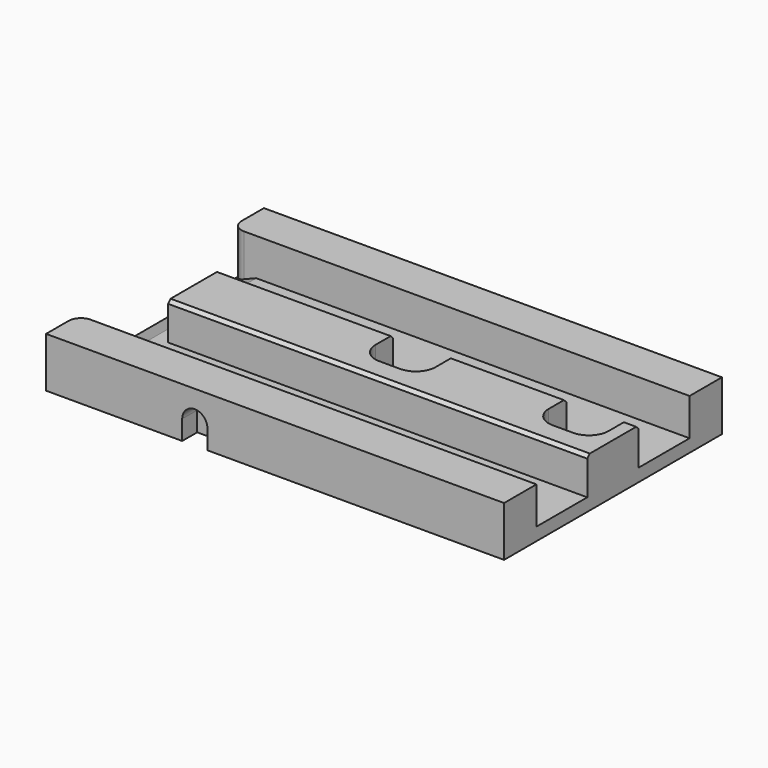
from build123d import *

# Parameters (mm, degrees)
F0_W      = 185.72
F0_H      = 110.42
F1_DEPTH  = 5.2
F3_DEPTH  = 110.42
F4_W      = 185.72
F4_H      = 16.4
F5_DEPTH  = 20.3
F6_W      = 24.4
F6_H      = 17
F6_W_2    = 24.3
F7_DEPTH  = 15.1
F8_R      = 8
F9_R      = 8
F10_R     = 5
F11_SIZE  = 1.3
F14_DEPTH = 7.6
F16_DEPTH = 7.6
F17_DEPTH = 20.301


with BuildPart() as f1:
    # F0 (on Top) → F1 (new body)
    with BuildSketch(Plane.XY):
        with Locations((-8.2149282098, -9.908063139)):
            Rectangle(F0_W, F0_H)
    extrude(amount=F1_DEPTH)

    # F2 (on face) → F3 (cut, through all)
    with BuildSketch(Plane.XZ.offset(65.118063139)):
        Polygon((-91.0749282098, 5.2), (-101.0749282098, 5.2), (-101.0749282098, 1.2), align=None)
    extrude(amount=-F3_DEPTH, mode=Mode.SUBTRACT)

    # F4 (on face) → F5 (join)
    with BuildSketch(Plane(origin=(0, 0, 0), x_dir=(1, 0, 0), z_dir=(0, 0, -1))):
        with Locations((-8.2149282098, 56.918063139)):
            Rectangle(F4_W, F4_H)
        with Locations((-8.2149282098, -37.101936861)):
            Rectangle(F4_W, F4_H)
        Polygon((84.6450717902, 9.908063139), (84.6450717902, 22.958063139), (-85.3549282098, 22.958063139), (-85.3549282098, 9.908063139), (-85.3549282098, -3.141936861), (84.6450717902, -3.141936861), align=None)
    extrude(amount=-F5_DEPTH)

    # F6 (on face) → F7 (cut)
    with BuildSketch(Plane.XY.offset(20.3)):
        with Locations((-2.7149282098, -5.358063139)):
            Rectangle(F6_W, F6_H)
        with Locations((67.4950717902, -5.358063139)):
            Rectangle(F6_W_2, F6_H)
    extrude(amount=-F7_DEPTH, mode=Mode.SUBTRACT)

    # F8
    f8_edges = [f1.edges().sort_by_distance(p)[0] for p in [
        (-14.914928, -13.858063, 12.75),
    ]]
    fillet(f8_edges, radius=F8_R)

    # F9
    f9_edges = [f1.edges().sort_by_distance(p)[0] for p in [
        (9.485072, -13.858063, 12.75),
        (79.645072, -13.858063, 12.75),
        (55.345072, -13.858063, 12.75),
    ]]
    fillet(f9_edges, radius=F9_R)

    # F10
    f10_edges = [f1.edges().sort_by_distance(p)[0] for p in [
        (-101.074928, 28.901937, 10.75),
        (-101.074928, -48.718063, 10.75),
    ]]
    fillet(f10_edges, radius=F10_R)

    # F11
    f11_edges = [f1.edges().sort_by_distance(p)[0] for p in [
        (-50.134928, 3.141937, 20.3),
        (32.415072, 3.141937, 20.3),
        (82.145072, 3.141937, 20.3),
        (-0.354928, -22.958063, 20.3),
    ]]
    chamfer(f11_edges, length=F11_SIZE)

    # F13 (on face) → F14 (cut)
    with BuildSketch(Plane.XZ.offset(65.118063139)):
        with BuildLine():
            Line((-45.8749282098, 7.9100113362), (-45.8749282098, 0))
            Line((-45.8749282098, 0), (-40.7749282098, 0))
            Line((-40.7749282098, 0), (-40.7749282098, 2.8100113362))
            ThreePointArc((-40.7749282098, 2.8100113362), (-44.3811727938, 4.3037667522), (-45.8749282098, 7.9100113362))
        make_face()
        with BuildLine():
            Line((-40.7749282098, 2.8100113362), (-40.7749282098, 0))
            Line((-40.7749282098, 0), (-35.6749282098, 0))
            Line((-35.6749282098, 0), (-35.6749282098, 7.9100113362))
            ThreePointArc((-35.6749282098, 7.9100113362), (-37.1686836257, 4.3037667522), (-40.7749282098, 2.8100113362))
        make_face()
        with BuildLine():
            Line((-40.7749282098, 7.9100113362), (-45.8749282098, 7.9100113362))
            ThreePointArc((-45.8749282098, 7.9100113362), (-44.3811727938, 4.3037667522), (-40.7749282098, 2.8100113362))
            Line((-40.7749282098, 2.8100113362), (-40.7749282098, 7.9100113362))
        make_face()
        with BuildLine():
            ThreePointArc((-35.6749282098, 7.9100113362), (-40.7749282098, 13.0100113362), (-45.8749282098, 7.9100113362))
            Line((-45.8749282098, 7.9100113362), (-40.7749282098, 7.9100113362))
            Line((-40.7749282098, 7.9100113362), (-35.6749282098, 7.9100113362))
        make_face()
        with BuildLine():
            Line((-40.7749282098, 7.9100113362), (-40.7749282098, 2.8100113362))
            ThreePointArc((-40.7749282098, 2.8100113362), (-37.1686836257, 4.3037667522), (-35.6749282098, 7.9100113362))
            Line((-35.6749282098, 7.9100113362), (-40.7749282098, 7.9100113362))
        make_face()
    extrude(amount=-F14_DEPTH, mode=Mode.SUBTRACT)

    # F15 (on face) → F16 (cut)
    with BuildSketch(Plane(origin=(0, 45.301936861, 0), x_dir=(-1, 0, 0), z_dir=(0, 1, 0))):
        with BuildLine():
            Line((40.7749282098, 0), (45.8749282098, 0))
            Line((45.8749282098, 0), (45.8749282098, 7.9))
            ThreePointArc((45.8749282098, 7.9), (44.3811727938, 4.2937554159), (40.7749282098, 2.8))
            Line((40.7749282098, 2.8), (40.7749282098, 0))
        make_face()
        with BuildLine():
            Line((35.6749282098, 0), (40.7749282098, 0))
            Line((40.7749282098, 0), (40.7749282098, 2.8))
            ThreePointArc((40.7749282098, 2.8), (37.1686836257, 4.2937554159), (35.6749282098, 7.9))
            Line((35.6749282098, 7.9), (35.6749282098, 0))
        make_face()
        with BuildLine():
            ThreePointArc((40.7749282098, 2.8), (44.3811727938, 4.2937554159), (45.8749282098, 7.9))
            Line((45.8749282098, 7.9), (40.7749282098, 7.9))
            Line((40.7749282098, 7.9), (40.7749282098, 2.8))
        make_face()
        with BuildLine():
            ThreePointArc((35.6749282098, 7.9), (37.1686836257, 4.2937554159), (40.7749282098, 2.8))
            Line((40.7749282098, 2.8), (40.7749282098, 7.9))
            Line((40.7749282098, 7.9), (35.6749282098, 7.9))
        make_face()
        with BuildLine():
            Line((40.7749282098, 7.9), (45.8749282098, 7.9))
            ThreePointArc((45.8749282098, 7.9), (40.7749282098, 13), (35.6749282098, 7.9))
            Line((35.6749282098, 7.9), (40.7749282098, 7.9))
        make_face()
    extrude(amount=-F16_DEPTH, mode=Mode.SUBTRACT)

    # F12 (on face) → F17 (cut, through all)
    with BuildSketch(Plane(origin=(0, 0, 0), x_dir=(1, 0, 0), z_dir=(0, 0, -1))):
        with BuildLine():
            ThreePointArc((-0.9549282098, -1.951936861), (1.9795649321, -0.7364300029), (3.1950717902, 2.198063139))
            Line((3.1950717902, 2.198063139), (-0.7049282098, 2.198063139))
            ThreePointArc((-0.7049282098, 2.198063139), (-1.2971901643, 0.0614770771), (-2.9049282098, -1.4652686778))
            ThreePointArc((-2.9049282098, -1.4652686778), (-1.9598344144, -1.8284320516), (-0.9549282098, -1.951936861))
        make_face()
        with BuildLine():
            Line((-0.7049282098, 2.198063139), (3.1950717902, 2.198063139))
            ThreePointArc((3.1950717902, 2.198063139), (1.9795649321, 5.132556281), (-0.9549282098, 6.348063139))
            ThreePointArc((-0.9549282098, 6.348063139), (-1.9598344144, 6.2245583296), (-2.9049282098, 5.8613949558))
            ThreePointArc((-2.9049282098, 5.8613949558), (-1.2971901643, 4.334649201), (-0.7049282098, 2.198063139))
        make_face()
        with BuildLine():
            ThreePointArc((69.0750717902, -1.951936861), (72.0095649321, -0.7364300029), (73.2250717902, 2.198063139))
            Line((73.2250717902, 2.198063139), (69.3250717902, 2.198063139))
            ThreePointArc((69.3250717902, 2.198063139), (68.7328098357, 0.0614770771), (67.1250717902, -1.4652686778))
            ThreePointArc((67.1250717902, -1.4652686778), (68.0701655856, -1.8284320516), (69.0750717902, -1.951936861))
        make_face()
        with BuildLine():
            Line((69.3250717902, 2.198063139), (73.2250717902, 2.198063139))
            ThreePointArc((73.2250717902, 2.198063139), (72.0095649321, 5.132556281), (69.0750717902, 6.348063139))
            ThreePointArc((69.0750717902, 6.348063139), (68.0701655856, 6.2245583296), (67.1250717902, 5.8613949558))
            ThreePointArc((67.1250717902, 5.8613949558), (68.7328098357, 4.334649201), (69.3250717902, 2.198063139))
        make_face()
        with BuildLine():
            ThreePointArc((67.1250717902, -1.4652686778), (68.7328098357, 0.0614770771), (69.3250717902, 2.198063139))
            Line((69.3250717902, 2.198063139), (69.0750717902, 2.198063139))
            Line((69.0750717902, 2.198063139), (65.1750717902, 2.198063139))
            Line((65.1750717902, 2.198063139), (64.9250717902, 2.198063139))
            ThreePointArc((64.9250717902, 2.198063139), (65.5173337448, 0.0614770771), (67.1250717902, -1.4652686778))
        make_face()
        with BuildLine():
            Line((69.0750717902, 2.198063139), (69.3250717902, 2.198063139))
            ThreePointArc((69.3250717902, 2.198063139), (68.7328098357, 4.334649201), (67.1250717902, 5.8613949558))
            ThreePointArc((67.1250717902, 5.8613949558), (65.5173337448, 4.334649201), (64.9250717902, 2.198063139))
            Line((64.9250717902, 2.198063139), (65.1750717902, 2.198063139))
            Line((65.1750717902, 2.198063139), (69.0750717902, 2.198063139))
        make_face()
        with BuildLine():
            ThreePointArc((67.1250717902, 5.8613949558), (68.0701655856, 6.2245583296), (69.0750717902, 6.348063139))
            Line((69.0750717902, 6.348063139), (65.1750717902, 6.348063139))
            ThreePointArc((65.1750717902, 6.348063139), (66.1799779949, 6.2245583296), (67.1250717902, 5.8613949558))
        make_face()
        with BuildLine():
            Line((65.1750717902, -1.951936861), (69.0750717902, -1.951936861))
            ThreePointArc((69.0750717902, -1.951936861), (68.0701655856, -1.8284320516), (67.1250717902, -1.4652686778))
            ThreePointArc((67.1250717902, -1.4652686778), (66.1799779949, -1.8284320516), (65.1750717902, -1.951936861))
        make_face()
        with BuildLine():
            ThreePointArc((64.9250717902, 2.198063139), (65.5173337448, 4.334649201), (67.1250717902, 5.8613949558))
            ThreePointArc((67.1250717902, 5.8613949558), (66.1799779949, 6.2245583296), (65.1750717902, 6.348063139))
            ThreePointArc((65.1750717902, 6.348063139), (62.2405786483, 5.132556281), (61.0250717902, 2.198063139))
            Line((61.0250717902, 2.198063139), (64.9250717902, 2.198063139))
        make_face()
        with BuildLine():
            ThreePointArc((65.1750717902, -1.951936861), (66.1799779949, -1.8284320516), (67.1250717902, -1.4652686778))
            ThreePointArc((67.1250717902, -1.4652686778), (65.5173337448, 0.0614770771), (64.9250717902, 2.198063139))
            Line((64.9250717902, 2.198063139), (61.0250717902, 2.198063139))
            ThreePointArc((61.0250717902, 2.198063139), (62.2405786483, -0.7364300029), (65.1750717902, -1.951936861))
        make_face()
        with BuildLine():
            ThreePointArc((-2.9049282098, -1.4652686778), (-1.2971901643, 0.0614770771), (-0.7049282098, 2.198063139))
            ThreePointArc((-0.7049282098, 2.198063139), (-1.2971901643, 4.334649201), (-2.9049282098, 5.8613949558))
            ThreePointArc((-2.9049282098, 5.8613949558), (-5.1049282098, 2.198063139), (-2.9049282098, -1.4652686778))
        make_face()
        with BuildLine():
            ThreePointArc((-2.9049282098, 5.8613949558), (-1.9598344144, 6.2245583296), (-0.9549282098, 6.348063139))
            Line((-0.9549282098, 6.348063139), (-4.8549282098, 6.348063139))
            ThreePointArc((-4.8549282098, 6.348063139), (-3.8500220051, 6.2245583296), (-2.9049282098, 5.8613949558))
        make_face()
        with BuildLine():
            Line((-4.8549282098, -1.951936861), (-0.9549282098, -1.951936861))
            ThreePointArc((-0.9549282098, -1.951936861), (-1.9598344144, -1.8284320516), (-2.9049282098, -1.4652686778))
            ThreePointArc((-2.9049282098, -1.4652686778), (-3.8500220051, -1.8284320516), (-4.8549282098, -1.951936861))
        make_face()
        with BuildLine():
            ThreePointArc((-2.9049282098, -1.4652686778), (-5.1049282098, 2.198063139), (-2.9049282098, 5.8613949558))
            ThreePointArc((-2.9049282098, 5.8613949558), (-3.8500220051, 6.2245583296), (-4.8549282098, 6.348063139))
            ThreePointArc((-4.8549282098, 6.348063139), (-9.0049282098, 2.198063139), (-4.8549282098, -1.951936861))
            ThreePointArc((-4.8549282098, -1.951936861), (-3.8500220051, -1.8284320516), (-2.9049282098, -1.4652686778))
        make_face()
    extrude(amount=-F17_DEPTH, mode=Mode.SUBTRACT)


solid = f1.part
